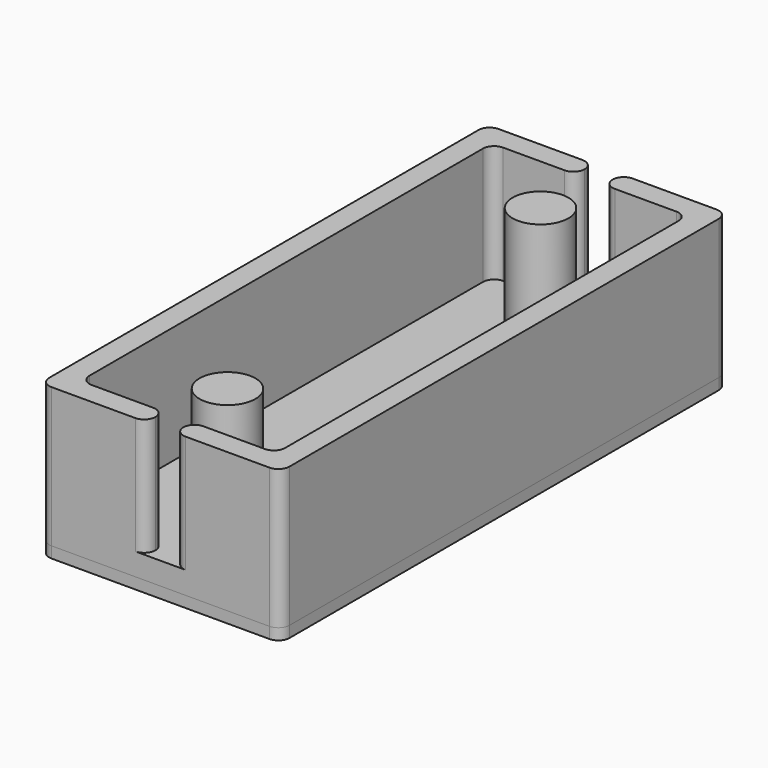
from build123d import *

# Parameters (mm, degrees)
F0_W     = 43
F0_H     = 100
F1_DEPTH = 25
F2_T     = -4
F3_R     = 5
F4_DEPTH = 21
F5_W     = 5
F5_H     = 10
F5_H_2   = 8
F6_DEPTH = 21
F7_R     = 1.99999
F8_DEPTH = 2


# Not quite as in the source:
# - a fillet or chamfer is up to 0.001 mm smaller than in the source, because OpenCascade refuses the exact size


with BuildPart() as f1:
    # F0 (on Top) → F1 (new body)
    with BuildSketch(Plane.XY):
        Rectangle(F0_W, F0_H)
    extrude(amount=F1_DEPTH)

    # F2
    f2_openings = [f1.faces().sort_by_distance(p)[0] for p in [
        (0, 0, 25),
    ]]
    offset(amount=F2_T, openings=f2_openings)

    # F3 (on face) → F4 (join, through all)
    with BuildSketch(Plane.XY.offset(4)):
        with Locations((0, 35)):
            Circle(F3_R)
        with Locations((0, -35)):
            Circle(F3_R)
    extrude(amount=F4_DEPTH)

    # F5 (on face) → F6 (cut, through all)
    with BuildSketch(Plane.XY.offset(25)):
        with Locations((0, 46)):
            Rectangle(F5_W, F5_H)
        with Locations((0, -46)):
            Rectangle(F5_W, F5_H_2)
    extrude(amount=-F6_DEPTH, mode=Mode.SUBTRACT)

    # F7 (radius 2 in the source; OpenCascade refuses exactly that, so slightly less here)
    f7_edges = [f1.edges().sort_by_distance(p)[0] for p in [
        (-2.5, -46, 14.5),
        (-2.5, -50, 14.5),
        (2.5, -50, 14.5),
        (-2.5, 50, 14.5),
        (-2.5, 46, 14.5),
        (2.5, 46, 14.5),
        (2.5, -46, 14.5),
        (2.5, 50, 14.5),
        (17.5, 46, 14.5),
        (17.5, -46, 14.5),
        (-17.5, -46, 14.5),
        (-17.5, 46, 14.5),
        (-21.5, -50, 12.5),
        (21.5, -50, 12.5),
        (21.5, 50, 12.5),
        (-21.5, 50, 12.5),
    ]]
    fillet(f7_edges, radius=F7_R)


with BuildPart() as f8:
    # F8 (new): a face of the model
    f8_faces = [f1.part.faces().sort_by_distance(p)[0] for p in [
        (0, 0, 0),
    ]]
    extrude(f8_faces, amount=F8_DEPTH)


solid = Compound([f1.part, f8.part])
